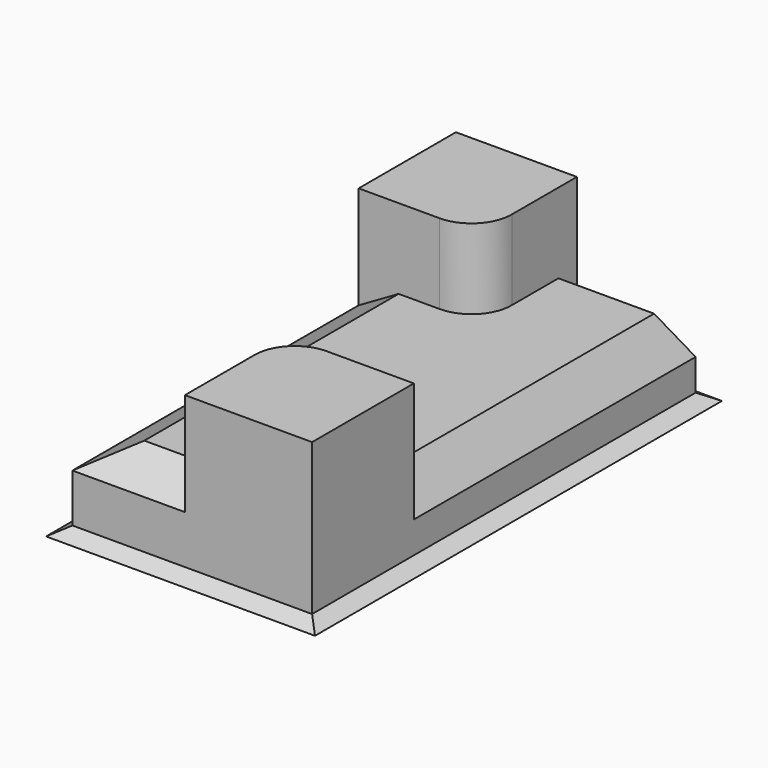
from build123d import *

# Parameters (mm, degrees)
F0_W          = 88.9
F0_H          = 165.1
F1_DEPTH      = 6.35
F2_DEPTH      = 25.4
F3_DEPTH      = 25.4
F4_T1_DEPTH   = 141.911978168
F4_T3_DEPTH   = 218.111978168
F4_T8_DEPTH   = 154.611978168
F4_T14_DEPTH  = 154.611978168
F4_T20_DEPTH  = 154.611978168
F4_T27_DEPTH  = 154.611978168
F4_T33_DEPTH  = 154.611978168
F4_T39_DEPTH  = 230.811978168
F4_T45_DEPTH  = 230.811978168
F4_T51_DEPTH  = 230.811978168
F4_T58_DEPTH  = 230.811978168
F4_T64_DEPTH  = 230.811978168
F4_T70_DEPTH  = 230.811978168
F4_T76_DEPTH  = 230.811978168
F4_T82_DEPTH  = 230.811978168
F4_T89_DEPTH  = 230.811978168
F4_T95_DEPTH  = 230.811978168
F4_T101_DEPTH = 154.611978168
F4_T107_DEPTH = 154.611978168
F4_T113_DEPTH = 154.611978168
F4_T120_DEPTH = 154.611978168
F4_T126_DEPTH = 154.611978168
F5_DEPTH      = 50.8


# Not quite as in the source:
# - a fillet or chamfer that OpenCascade refuses, or shapes differently, is made with other operations: its cross-section is extruded or revolved along the edge and cut away or added


with BuildPart() as f1:
    # F0 (on Top) → F1 (new body)
    with BuildSketch(Plane.XY):
        with Locations((9.5230986749, 3.1729897651)):
            Rectangle(F0_W, F0_H)
        Polygon((-28.5769013251, 40.7291018275), (-28.5769013251, 79.3729897651), (9.8754219143, 79.3729897651), (47.6230986749, 79.3729897651), (47.6230986749, -32.5965460718), (47.6230986749, -73.0270102349), (7.1926345117, -73.0270102349), (-28.5769013251, -73.0270102349), align=None, mode=Mode.SUBTRACT)
    extrude(amount=F1_DEPTH)

    # F0 (on Top) → F2 (join)
    with BuildSketch(Plane.XY):
        with BuildLine():
            Line((47.6230986749, 79.3729897651), (9.8754219143, 79.3729897651))
            Line((9.8754219143, 79.3729897651), (9.8754219143, 53.6192430722))
            ThreePointArc((9.8754219143, 53.6192430722), (6.2240768174, 44.5163243089), (-2.8231546322, 40.7291018275))
            Line((-2.8231546322, 40.7291018275), (-28.5769013251, 40.7291018275))
            Line((-28.5769013251, 40.7291018275), (-28.5769013251, -73.0270102349))
            Line((-28.5769013251, -73.0270102349), (7.1926345117, -73.0270102349))
            Line((7.1926345117, -73.0270102349), (7.1926345117, -45.2965460718))
            ThreePointArc((7.1926345117, -45.2965460718), (10.9123783907, -36.3162899507), (19.8926345117, -32.5965460718))
            Line((19.8926345117, -32.5965460718), (47.6230986749, -32.5965460718))
            Line((47.6230986749, -32.5965460718), (47.6230986749, 79.3729897651))
        make_face()
    extrude(amount=F2_DEPTH)

    # F0 (on Top) → F3 (join)
    with BuildSketch(Plane.XY):
        with BuildLine():
            Line((9.8754219143, 79.3729897651), (-28.5769013251, 79.3729897651))
            Line((-28.5769013251, 79.3729897651), (-28.5769013251, 40.7291018275))
            Line((-28.5769013251, 40.7291018275), (-2.8231546322, 40.7291018275))
            ThreePointArc((-2.8231546322, 40.7291018275), (6.2240768174, 44.5163243089), (9.8754219143, 53.6192430722))
            Line((9.8754219143, 53.6192430722), (9.8754219143, 79.3729897651))
        make_face()
        with BuildLine():
            Line((47.6230986749, -73.0270102349), (47.6230986749, -32.5965460718))
            Line((47.6230986749, -32.5965460718), (19.8926345117, -32.5965460718))
            ThreePointArc((19.8926345117, -32.5965460718), (10.9123783907, -36.3162899507), (7.1926345117, -45.2965460718))
            Line((7.1926345117, -45.2965460718), (7.1926345117, -73.0270102349))
            Line((7.1926345117, -73.0270102349), (47.6230986749, -73.0270102349))
        make_face()
    extrude(amount=F3_DEPTH)

    # F4: chamfer of 12.7 x 7.3323484187 on 8 edges, made by hand

    # F4_s2 → F4_t1 (cut)
    with BuildSketch(Plane.YZ.offset(-61.4328904091)):
        Polygon((-73.0270102349, 18.0676515813), (-60.3270102349, 25.4), (-73.0270102349, 25.4), align=None)
        Polygon((72.0406413464, 25.4), (79.3729897651, 12.7), (79.3729897651, 25.4), align=None)
    extrude(amount=F4_T1_DEPTH, mode=Mode.SUBTRACT)

    # F4_s4 → F4_t3 (cut)
    with BuildSketch(Plane.XZ.offset(-112.2289788491)):
        Polygon((-15.8769013251, 25.4), (-28.5769013251, 18.0676515813), (-28.5769013251, 25.4), align=None)
        Polygon((40.2907502562, 25.4), (47.6230986749, 12.7), (47.6230986749, 25.4), align=None)
    extrude(amount=F4_T3_DEPTH, mode=Mode.SUBTRACT)


with BuildPart() as f4_tool6:
    # F4_s7 → F4_t8 (new body)
    with BuildSketch(Plane.YZ.offset(-67.7828904091)):
        Polygon((-66.6770102349, 6.35), (-79.3770102349, -0.9823484187), (-79.3770102349, 6.35), align=None)
    extrude(amount=F4_T8_DEPTH)

    split(bisect_by=Plane.YZ.offset(-28.5769013251), keep=Keep.BOTTOM)

    split(bisect_by=Plane.XZ.offset(73.0270102349), keep=Keep.BOTTOM)


with BuildPart() as f1_1:
    add(f1.part)

    # F4_t5: cut F4_tool6
    add(f4_tool6.part, mode=Mode.SUBTRACT)


with BuildPart() as f4_tool12:
    # F4_s13 → F4_t14 (new body)
    with BuildSketch(Plane.YZ.offset(-67.7828904091)):
        Polygon((-66.6770102349, 6.35), (-79.3770102349, -0.9823484187), (-79.3770102349, 6.35), align=None)
    extrude(amount=F4_T14_DEPTH)

    split(bisect_by=Plane.YZ.offset(-28.5769013251), keep=Keep.BOTTOM)

    split(bisect_by=Plane.XZ.offset(73.0270102349), keep=Keep.TOP)


with BuildPart() as f1_2:
    add(f1_1.part)

    # F4_t11: cut F4_tool12
    add(f4_tool12.part, mode=Mode.SUBTRACT)


with BuildPart() as f4_tool18:
    # F4_s19 → F4_t20 (new body)
    with BuildSketch(Plane.YZ.offset(-67.7828904091)):
        Polygon((-66.6770102349, 6.35), (-79.3770102349, -0.9823484187), (-79.3770102349, 6.35), align=None)
    extrude(amount=F4_T20_DEPTH)

    split(bisect_by=Plane.YZ.offset(-28.5769013251), keep=Keep.TOP)

    split(bisect_by=Plane.YZ.offset(47.6230986749), keep=Keep.BOTTOM)

    split(bisect_by=Plane.XZ.offset(73.0270102349), keep=Keep.TOP)


with BuildPart() as f1_3:
    add(f1_2.part)

    # F4_t17: cut F4_tool18
    add(f4_tool18.part, mode=Mode.SUBTRACT)


with BuildPart() as f4_tool25:
    # F4_s26 → F4_t27 (new body)
    with BuildSketch(Plane.YZ.offset(-67.7828904091)):
        Polygon((-66.6770102349, 6.35), (-79.3770102349, -0.9823484187), (-79.3770102349, 6.35), align=None)
    extrude(amount=F4_T27_DEPTH)

    split(bisect_by=Plane.YZ.offset(47.6230986749), keep=Keep.TOP)

    split(bisect_by=Plane.XZ.offset(73.0270102349), keep=Keep.BOTTOM)


with BuildPart() as f1_4:
    add(f1_3.part)

    # F4_t24: cut F4_tool25
    add(f4_tool25.part, mode=Mode.SUBTRACT)


with BuildPart() as f4_tool31:
    # F4_s32 → F4_t33 (new body)
    with BuildSketch(Plane.YZ.offset(-67.7828904091)):
        Polygon((-66.6770102349, 6.35), (-79.3770102349, -0.9823484187), (-79.3770102349, 6.35), align=None)
    extrude(amount=F4_T33_DEPTH)

    split(bisect_by=Plane.YZ.offset(47.6230986749), keep=Keep.TOP)

    split(bisect_by=Plane.XZ.offset(73.0270102349), keep=Keep.TOP)


with BuildPart() as f1_5:
    add(f1_4.part)

    # F4_t30: cut F4_tool31
    add(f4_tool31.part, mode=Mode.SUBTRACT)


with BuildPart() as f4_tool37:
    # F4_s38 → F4_t39 (new body)
    with BuildSketch(Plane.XZ.offset(112.2329993189)):
        Polygon((41.2730986749, 6.35), (53.9730986749, -0.9823484187), (53.9730986749, 6.35), align=None)
    extrude(amount=-F4_T39_DEPTH)

    split(bisect_by=Plane.YZ.offset(47.6230986749), keep=Keep.BOTTOM)

    split(bisect_by=Plane.XZ.offset(73.0270102349), keep=Keep.TOP)


with BuildPart() as f1_6:
    add(f1_5.part)

    # F4_t36: cut F4_tool37
    add(f4_tool37.part, mode=Mode.SUBTRACT)


with BuildPart() as f4_tool43:
    # F4_s44 → F4_t45 (new body)
    with BuildSketch(Plane.XZ.offset(112.2329993189)):
        Polygon((41.2730986749, 6.35), (53.9730986749, -0.9823484187), (53.9730986749, 6.35), align=None)
    extrude(amount=-F4_T45_DEPTH)

    split(bisect_by=Plane.YZ.offset(47.6230986749), keep=Keep.TOP)

    split(bisect_by=Plane.XZ.offset(73.0270102349), keep=Keep.TOP)


with BuildPart() as f1_7:
    add(f1_6.part)

    # F4_t42: cut F4_tool43
    add(f4_tool43.part, mode=Mode.SUBTRACT)


with BuildPart() as f4_tool49:
    # F4_s50 → F4_t51 (new body)
    with BuildSketch(Plane.XZ.offset(112.2329993189)):
        Polygon((41.2730986749, 6.35), (53.9730986749, -0.9823484187), (53.9730986749, 6.35), align=None)
    extrude(amount=-F4_T51_DEPTH)

    split(bisect_by=Plane.XZ.offset(-79.3729897651), keep=Keep.TOP)

    split(bisect_by=Plane.YZ.offset(47.6230986749), keep=Keep.TOP)

    split(bisect_by=Plane.XZ.offset(73.0270102349), keep=Keep.BOTTOM)


with BuildPart() as f1_8:
    add(f1_7.part)

    # F4_t48: cut F4_tool49
    add(f4_tool49.part, mode=Mode.SUBTRACT)


with BuildPart() as f4_tool56:
    # F4_s57 → F4_t58 (new body)
    with BuildSketch(Plane.XZ.offset(112.2329993189)):
        Polygon((41.2730986749, 6.35), (53.9730986749, -0.9823484187), (53.9730986749, 6.35), align=None)
    extrude(amount=-F4_T58_DEPTH)

    split(bisect_by=Plane.XZ.offset(-79.3729897651), keep=Keep.BOTTOM)

    split(bisect_by=Plane.YZ.offset(47.6230986749), keep=Keep.BOTTOM)


with BuildPart() as f1_9:
    add(f1_8.part)

    # F4_t55: cut F4_tool56
    add(f4_tool56.part, mode=Mode.SUBTRACT)


with BuildPart() as f4_tool62:
    # F4_s63 → F4_t64 (new body)
    with BuildSketch(Plane.XZ.offset(112.2329993189)):
        Polygon((41.2730986749, 6.35), (53.9730986749, -0.9823484187), (53.9730986749, 6.35), align=None)
    extrude(amount=-F4_T64_DEPTH)

    split(bisect_by=Plane.XZ.offset(-79.3729897651), keep=Keep.BOTTOM)

    split(bisect_by=Plane.YZ.offset(47.6230986749), keep=Keep.TOP)


with BuildPart() as f1_10:
    add(f1_9.part)

    # F4_t61: cut F4_tool62
    add(f4_tool62.part, mode=Mode.SUBTRACT)


with BuildPart() as f4_tool68:
    # F4_s69 → F4_t70 (new body)
    with BuildSketch(Plane.XZ.offset(-118.5789788491)):
        Polygon((-22.2269013251, 6.35), (-34.9269013251, -0.9823484187), (-34.9269013251, 6.35), align=None)
    extrude(amount=F4_T70_DEPTH)

    split(bisect_by=Plane.YZ.offset(-28.5769013251), keep=Keep.TOP)

    split(bisect_by=Plane.XZ.offset(-79.3729897651), keep=Keep.BOTTOM)


with BuildPart() as f1_11:
    add(f1_10.part)

    # F4_t67: cut F4_tool68
    add(f4_tool68.part, mode=Mode.SUBTRACT)


with BuildPart() as f4_tool74:
    # F4_s75 → F4_t76 (new body)
    with BuildSketch(Plane.XZ.offset(-118.5789788491)):
        Polygon((-22.2269013251, 6.35), (-34.9269013251, -0.9823484187), (-34.9269013251, 6.35), align=None)
    extrude(amount=F4_T76_DEPTH)

    split(bisect_by=Plane.YZ.offset(-28.5769013251), keep=Keep.BOTTOM)

    split(bisect_by=Plane.XZ.offset(-79.3729897651), keep=Keep.BOTTOM)


with BuildPart() as f1_12:
    add(f1_11.part)

    # F4_t73: cut F4_tool74
    add(f4_tool74.part, mode=Mode.SUBTRACT)


with BuildPart() as f4_tool80:
    # F4_s81 → F4_t82 (new body)
    with BuildSketch(Plane.XZ.offset(-118.5789788491)):
        Polygon((-22.2269013251, 6.35), (-34.9269013251, -0.9823484187), (-34.9269013251, 6.35), align=None)
    extrude(amount=F4_T82_DEPTH)

    split(bisect_by=Plane.YZ.offset(-28.5769013251), keep=Keep.BOTTOM)

    split(bisect_by=Plane.XZ.offset(-79.3729897651), keep=Keep.TOP)

    split(bisect_by=Plane.XZ.offset(73.0270102349), keep=Keep.BOTTOM)


with BuildPart() as f1_13:
    add(f1_12.part)

    # F4_t79: cut F4_tool80
    add(f4_tool80.part, mode=Mode.SUBTRACT)


with BuildPart() as f4_tool87:
    # F4_s88 → F4_t89 (new body)
    with BuildSketch(Plane.XZ.offset(-118.5789788491)):
        Polygon((-22.2269013251, 6.35), (-34.9269013251, -0.9823484187), (-34.9269013251, 6.35), align=None)
    extrude(amount=F4_T89_DEPTH)

    split(bisect_by=Plane.YZ.offset(-28.5769013251), keep=Keep.TOP)

    split(bisect_by=Plane.XZ.offset(73.0270102349), keep=Keep.TOP)


with BuildPart() as f1_14:
    add(f1_13.part)

    # F4_t86: cut F4_tool87
    add(f4_tool87.part, mode=Mode.SUBTRACT)


with BuildPart() as f4_tool93:
    # F4_s94 → F4_t95 (new body)
    with BuildSketch(Plane.XZ.offset(-118.5789788491)):
        Polygon((-22.2269013251, 6.35), (-34.9269013251, -0.9823484187), (-34.9269013251, 6.35), align=None)
    extrude(amount=F4_T95_DEPTH)

    split(bisect_by=Plane.YZ.offset(-28.5769013251), keep=Keep.BOTTOM)

    split(bisect_by=Plane.XZ.offset(73.0270102349), keep=Keep.TOP)


with BuildPart() as f1_15:
    add(f1_14.part)

    # F4_t92: cut F4_tool93
    add(f4_tool93.part, mode=Mode.SUBTRACT)


with BuildPart() as f4_tool99:
    # F4_s100 → F4_t101 (new body)
    with BuildSketch(Plane.YZ.offset(86.8290877589)):
        Polygon((85.7229897651, -0.9823484187), (73.0229897651, 6.35), (85.7229897651, 6.35), align=None)
    extrude(amount=-F4_T101_DEPTH)

    split(bisect_by=Plane.XZ.offset(-79.3729897651), keep=Keep.BOTTOM)

    split(bisect_by=Plane.YZ.offset(47.6230986749), keep=Keep.TOP)


with BuildPart() as f1_16:
    add(f1_15.part)

    # F4_t98: cut F4_tool99
    add(f4_tool99.part, mode=Mode.SUBTRACT)


with BuildPart() as f4_tool105:
    # F4_s106 → F4_t107 (new body)
    with BuildSketch(Plane.YZ.offset(86.8290877589)):
        Polygon((85.7229897651, -0.9823484187), (73.0229897651, 6.35), (85.7229897651, 6.35), align=None)
    extrude(amount=-F4_T107_DEPTH)

    split(bisect_by=Plane.XZ.offset(-79.3729897651), keep=Keep.TOP)

    split(bisect_by=Plane.YZ.offset(47.6230986749), keep=Keep.TOP)


with BuildPart() as f1_17:
    add(f1_16.part)

    # F4_t104: cut F4_tool105
    add(f4_tool105.part, mode=Mode.SUBTRACT)


with BuildPart() as f4_tool111:
    # F4_s112 → F4_t113 (new body)
    with BuildSketch(Plane.YZ.offset(86.8290877589)):
        Polygon((85.7229897651, -0.9823484187), (73.0229897651, 6.35), (85.7229897651, 6.35), align=None)
    extrude(amount=-F4_T113_DEPTH)

    split(bisect_by=Plane.YZ.offset(-28.5769013251), keep=Keep.TOP)

    split(bisect_by=Plane.XZ.offset(-79.3729897651), keep=Keep.BOTTOM)

    split(bisect_by=Plane.YZ.offset(47.6230986749), keep=Keep.BOTTOM)


with BuildPart() as f1_18:
    add(f1_17.part)

    # F4_t110: cut F4_tool111
    add(f4_tool111.part, mode=Mode.SUBTRACT)


with BuildPart() as f4_tool118:
    # F4_s119 → F4_t120 (new body)
    with BuildSketch(Plane.YZ.offset(86.8290877589)):
        Polygon((85.7229897651, -0.9823484187), (73.0229897651, 6.35), (85.7229897651, 6.35), align=None)
    extrude(amount=-F4_T120_DEPTH)

    split(bisect_by=Plane.YZ.offset(-28.5769013251), keep=Keep.BOTTOM)

    split(bisect_by=Plane.XZ.offset(-79.3729897651), keep=Keep.BOTTOM)


with BuildPart() as f1_19:
    add(f1_18.part)

    # F4_t117: cut F4_tool118
    add(f4_tool118.part, mode=Mode.SUBTRACT)


with BuildPart() as f4_tool124:
    # F4_s125 → F4_t126 (new body)
    with BuildSketch(Plane.YZ.offset(86.8290877589)):
        Polygon((85.7229897651, -0.9823484187), (73.0229897651, 6.35), (85.7229897651, 6.35), align=None)
    extrude(amount=-F4_T126_DEPTH)

    split(bisect_by=Plane.YZ.offset(-28.5769013251), keep=Keep.BOTTOM)

    split(bisect_by=Plane.XZ.offset(-79.3729897651), keep=Keep.TOP)


with BuildPart() as f1_20:
    add(f1_19.part)

    # F4_t123: cut F4_tool124
    add(f4_tool124.part, mode=Mode.SUBTRACT)

    # F0 (on Top) → F5 (join)
    with BuildSketch(Plane.XY):
        with BuildLine():
            Line((47.6230986749, -73.0270102349), (47.6230986749, -32.5965460718))
            Line((47.6230986749, -32.5965460718), (19.8926345117, -32.5965460718))
            ThreePointArc((19.8926345117, -32.5965460718), (10.9123783907, -36.3162899507), (7.1926345117, -45.2965460718))
            Line((7.1926345117, -45.2965460718), (7.1926345117, -73.0270102349))
            Line((7.1926345117, -73.0270102349), (47.6230986749, -73.0270102349))
        make_face()
        with BuildLine():
            Line((9.8754219143, 79.3729897651), (-28.5769013251, 79.3729897651))
            Line((-28.5769013251, 79.3729897651), (-28.5769013251, 40.7291018275))
            Line((-28.5769013251, 40.7291018275), (-2.8231546322, 40.7291018275))
            ThreePointArc((-2.8231546322, 40.7291018275), (6.2240768174, 44.5163243089), (9.8754219143, 53.6192430722))
            Line((9.8754219143, 53.6192430722), (9.8754219143, 79.3729897651))
        make_face()
    extrude(amount=F5_DEPTH)


solid = f1_20.part
